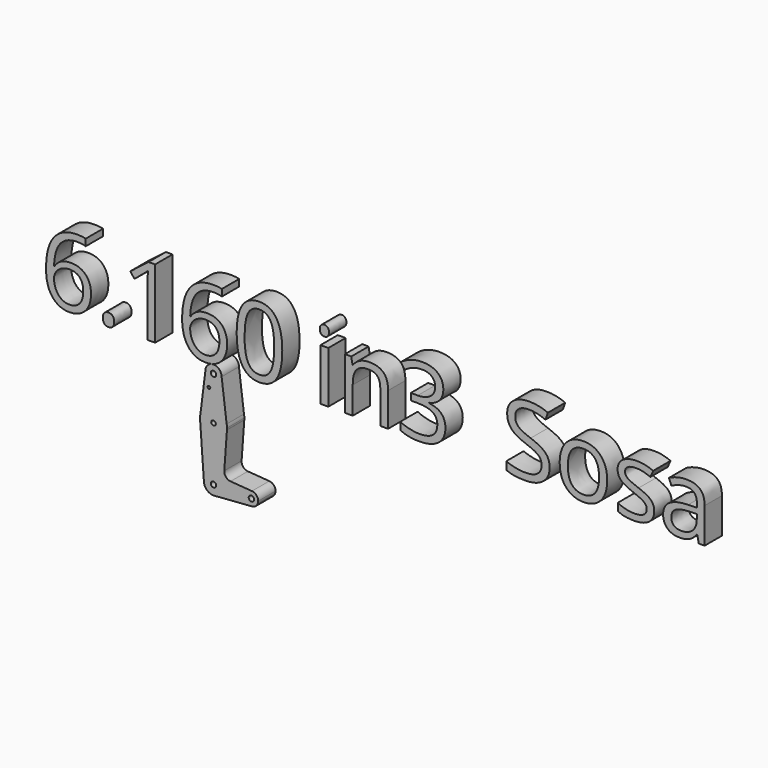
from build123d import *

# Parameters (mm, degrees)
F0_R         = 1.5875
F0_TEXT_SIZE = 113.1918022616
F1_DEPTH     = 25.4


# Not quite as in the source:
# - Text() gives the source's letters only with a copy of the font that has no kerning and outlines rounded to 1/6400 em; it was checked with that copy


with BuildPart() as f1:
    # F0 (on Front) → F1 (new body)
    with BuildSketch(Plane.XZ):
        with BuildLine():
            ThreePointArc((-400.7420838151, 176.1782964784), (-397.9522759059, 169.4431043876), (-391.2170838151, 166.6532964784))
            ThreePointArc((-391.2170838151, 166.6532964784), (-384.4818917243, 169.4431043876), (-381.6920838151, 176.1782964784))
            ThreePointArc((-381.6920838151, 176.1782964784), (-381.6920848779, 176.1827960369), (-381.6920880662, 176.1872955944))
            ThreePointArc((-381.6920880662, 176.1872955944), (-391.2215833736, 185.7032954156), (-400.7420838151, 176.1782964784))
        make_face()
        with BuildLine():
            ThreePointArc((-388.0420838151, 176.1782964784), (-388.9720197848, 173.9332324481), (-391.2170838151, 173.0032964784))
            ThreePointArc((-391.2170838151, 173.0032964784), (-393.4621478454, 178.4233605087), (-388.0420838151, 176.1782964784))
        make_face(mode=Mode.SUBTRACT)
        with BuildLine():
            ThreePointArc((-381.6920838151, 176.1782964784), (-384.4818917243, 169.4431043876), (-391.2170838151, 166.6532964784))
            Line((-391.2170838151, 166.6532964784), (-391.2170838151, 141.2532964784))
            ThreePointArc((-391.2170838151, 141.2532964784), (-381.4705044473, 137.9090512692), (-375.8303756442, 129.2853204945))
            Line((-375.8303756442, 129.2853204945), (-381.6920880662, 176.1872955944))
            ThreePointArc((-381.6920880662, 176.1872955944), (-381.6920848779, 176.1827960369), (-381.6920838151, 176.1782964784))
        make_face()
        with BuildLine():
            Line((-391.2170838151, 141.2532964784), (-391.2170838151, 166.6532964784))
            ThreePointArc((-391.2170838151, 166.6532964784), (-397.9522759059, 169.4431043876), (-400.7420838151, 176.1782964784))
            Line((-400.7420838151, 176.1782964784), (-406.6036222766, 129.2859887861))
            ThreePointArc((-406.6036222766, 129.2859887861), (-400.9633910546, 137.9092629292), (-391.2170838151, 141.2532964784))
        make_face()
        with Locations((-396.5730654791, 160.4091426542)):
            Circle(F0_R, mode=Mode.SUBTRACT)
        with BuildLine():
            ThreePointArc((-375.8303756442, 129.2853204945), (-381.4705044473, 137.9090512692), (-391.2170838151, 141.2532964784))
            Line((-391.2170838151, 141.2532964784), (-391.2170838151, 128.0530687261))
            ThreePointArc((-391.2170838151, 128.0530687261), (-389.3257342206, 127.2696460729), (-388.5423115674, 125.3782964784))
            ThreePointArc((-388.5423115674, 125.3782964784), (-389.3257342206, 123.4869468839), (-391.2170838151, 122.7035242307))
            Line((-391.2170838151, 122.7035242307), (-391.2170838151, 109.5032964784))
            ThreePointArc((-391.2170838151, 109.5032964784), (-380.7479513202, 113.4446092944), (-375.4771969135, 123.3115150856))
            Line((-375.4771969135, 123.3115150856), (-375.4594897165, 123.4511604622))
            ThreePointArc((-375.4594897165, 123.4511604622), (-375.3714624749, 124.4129419619), (-375.3420838151, 125.3782964784))
            Line((-375.3420838151, 125.3782964784), (-375.8303756442, 129.2853204945))
        make_face()
        with BuildLine():
            Line((-391.2170838151, 128.0530687261), (-391.2170838151, 141.2532964784))
            ThreePointArc((-391.2170838151, 141.2532964784), (-400.9633910546, 137.9092629292), (-406.6036222766, 129.2859887861))
            Line((-406.6036222766, 129.2859887861), (-407.0920838151, 125.3782964784))
            Line((-407.0920838151, 125.3782964784), (-406.9277330874, 123.0998925542))
            ThreePointArc((-406.9277330874, 123.0998925542), (-401.6056824382, 113.374436947), (-391.2170838151, 109.5032964784))
            Line((-391.2170838151, 109.5032964784), (-391.2170838151, 122.7035242307))
            ThreePointArc((-391.2170838151, 122.7035242307), (-393.8918560628, 125.3782964784), (-391.2170838151, 128.0530687261))
        make_face()
        with BuildLine():
            ThreePointArc((-375.8245854605, 129.2624462441), (-375.8274763024, 129.2738844451), (-375.8303756442, 129.2853204945))
            Line((-375.8303756442, 129.2853204945), (-375.3420838151, 125.3782964784))
            Line((-375.3420838151, 125.3782964784), (-375.8245854605, 129.2624462441))
        make_face()
        with BuildLine():
            Line((-407.0920838151, 125.3782964784), (-406.6036222766, 129.2859887861))
            ThreePointArc((-406.6036222766, 129.2859887861), (-406.9694951079, 127.34734789), (-407.0920838151, 125.3782964784))
        make_face()
        with BuildLine():
            ThreePointArc((-375.3420838151, 125.3782964784), (-375.4631710252, 127.3352984738), (-375.8245854605, 129.2624462441))
            Line((-375.8245854605, 129.2624462441), (-375.3420838151, 125.3782964784))
        make_face()
        with BuildLine():
            Line((-406.9277330874, 123.0998925542), (-407.0920838151, 125.3782964784))
            ThreePointArc((-407.0920838151, 125.3782964784), (-407.0509428235, 124.2361345368), (-406.9277330874, 123.0998925542))
        make_face()
        with BuildLine():
            ThreePointArc((-375.4771969135, 123.3115150856), (-380.7479513202, 113.4446092944), (-391.2170838151, 109.5032964784))
            Line((-391.2170838151, 109.5032964784), (-391.2170838151, 73.1435077203))
            ThreePointArc((-391.2170838151, 73.1435077203), (-383.2513765544, 69.8440037391), (-379.9518725731, 61.8782964784))
            Line((-379.9518725731, 61.8782964784), (-354.7045838151, 61.8782964784))
            ThreePointArc((-354.7045838151, 61.8782964784), (-352.1675998312, 67.6953690248), (-346.1783896708, 69.7939357738))
            Line((-346.1783896708, 69.7939357738), (-371.2596524852, 71.6592539386))
            ThreePointArc((-371.2596524852, 71.6592539386), (-376.6879135718, 74.3923107104), (-378.5994853619, 80.1613237138))
            Line((-378.5994853619, 80.1613237138), (-375.4771969135, 123.3115150856))
        make_face()
        with BuildLine():
            Line((-391.2170838151, 73.1435077203), (-391.2170838151, 109.5032964784))
            ThreePointArc((-391.2170838151, 109.5032964784), (-401.6056824382, 113.374436947), (-406.9277330874, 123.0998925542))
            Line((-406.9277330874, 123.0998925542), (-402.4531006028, 61.0677959716))
            ThreePointArc((-402.4531006028, 61.0677959716), (-399.4643695427, 69.552100128), (-391.2170838151, 73.1435077203))
        make_face()
        with BuildLine():
            ThreePointArc((-375.4771969135, 123.3115150856), (-375.4681885349, 123.3813181476), (-375.4594897165, 123.4511604622))
            Line((-375.4594897165, 123.4511604622), (-375.4771969135, 123.3115150856))
        make_face()
        with BuildLine():
            Line((-391.2170838151, 65.0532964784), (-391.2170838151, 73.1435077203))
            ThreePointArc((-391.2170838151, 73.1435077203), (-399.4643695427, 69.552100128), (-402.4531006028, 61.0677959716))
            ThreePointArc((-402.4531006028, 61.0677959716), (-398.8908874647, 53.6310107508), (-391.2170838151, 50.6130852364))
            Line((-391.2170838151, 50.6130852364), (-389.5477777947, 50.7374526263))
            ThreePointArc((-389.5477777947, 50.7374526263), (-382.6815677419, 54.5264293897), (-379.9518725731, 61.8782964784))
            Line((-379.9518725731, 61.8782964784), (-388.0420838151, 61.8782964784))
            ThreePointArc((-388.0420838151, 61.8782964784), (-393.4621478454, 59.6332324481), (-391.2170838151, 65.0532964784))
        make_face()
        with BuildLine():
            Line((-354.7045838151, 61.8782964784), (-379.9518725731, 61.8782964784))
            ThreePointArc((-379.9518725731, 61.8782964784), (-382.6815677419, 54.5264293897), (-389.5477777947, 50.7374526263))
            Line((-389.5477777947, 50.7374526263), (-346.4830599997, 53.9458796511))
            ThreePointArc((-346.4830599997, 53.9458796511), (-347.0731961151, 53.9467013356), (-347.6616401596, 53.9913658209))
            ThreePointArc((-347.6616401596, 53.9913658209), (-352.6875756542, 56.5913613896), (-354.7045838151, 61.8782964784))
        make_face()
        with BuildLine():
            Line((-389.5477777947, 50.7374526263), (-391.2170838151, 50.6130852364))
            ThreePointArc((-391.2170838151, 50.6130852364), (-390.3801175916, 50.6442201093), (-389.5477777947, 50.7374526263))
        make_face()
        with BuildLine():
            ThreePointArc((-346.1783896708, 69.7939357738), (-352.1675998312, 67.6953690248), (-354.7045838151, 61.8782964784))
            ThreePointArc((-354.7045838151, 61.8782964784), (-352.6875756542, 56.5913613896), (-347.6616401596, 53.9913658209))
            ThreePointArc((-347.6616401596, 53.9913658209), (-347.0731961151, 53.9467013356), (-346.4830599997, 53.9458796511))
            Line((-346.4830599997, 53.9458796511), (-345.8725274705, 53.9913658209))
            ThreePointArc((-345.8725274705, 53.9913658209), (-340.8465919759, 56.5913613896), (-338.8295838151, 61.8782964784))
            ThreePointArc((-338.8295838151, 61.8782964784), (-340.9500112687, 67.2788124945), (-346.1783896708, 69.7939357738))
        make_face()
        with BuildLine():
            ThreePointArc((-343.5920838151, 61.8782964784), (-346.7670838151, 58.7032964784), (-349.9420838151, 61.8782964784))
            ThreePointArc((-349.9420838151, 61.8782964784), (-346.7670838151, 65.0532964784), (-343.5920838151, 61.8782964784))
        make_face(mode=Mode.SUBTRACT)
        with BuildLine():
            Line((-345.8725274705, 53.9913658209), (-346.4830599997, 53.9458796511))
            ThreePointArc((-346.4830599997, 53.9458796511), (-346.1773550247, 53.9627341987), (-345.8725274705, 53.9913658209))
        make_face()
        with Locations((-593.9961671829, 185.9366632998)):
            Text('6.160 in3  Sosa', F0_TEXT_SIZE, font='Open Sans', text_align=(TextAlign.LEFT, TextAlign.BOTTOM))
        with BuildLine():
            ThreePointArc((-379.9518725731, 61.8782964784), (-383.2513765544, 69.8440037391), (-391.2170838151, 73.1435077203))
            Line((-391.2170838151, 73.1435077203), (-391.2170838151, 65.0532964784))
            ThreePointArc((-391.2170838151, 65.0532964784), (-388.9720197848, 64.1233605087), (-388.0420838151, 61.8782964784))
            Line((-388.0420838151, 61.8782964784), (-379.9518725731, 61.8782964784))
        make_face()
    extrude(amount=F1_DEPTH)


solid = f1.part
